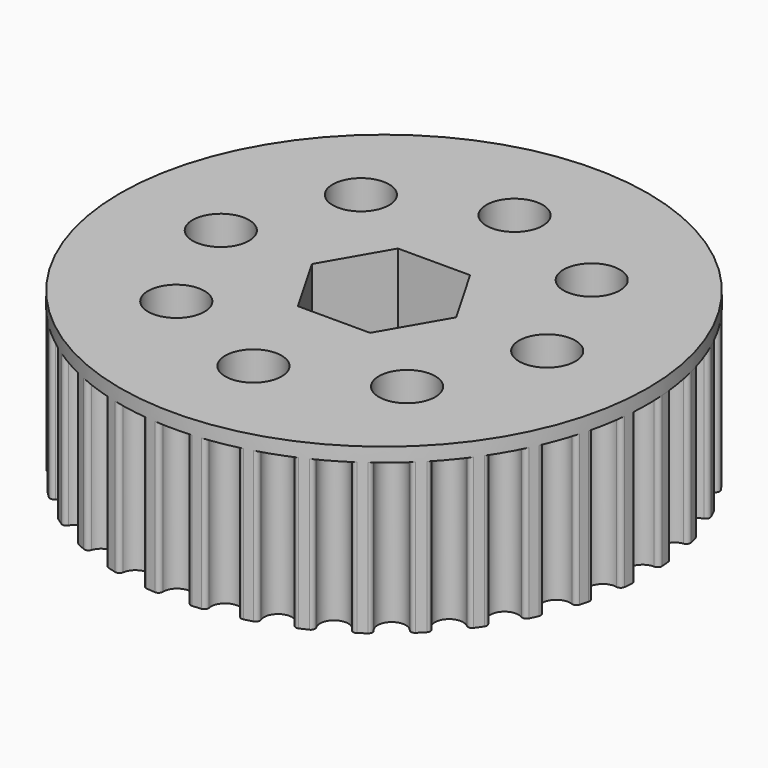
from build123d import *

# Parameters (mm, degrees)
F2_R            = 28.0753897893
F3_DEPTH        = 16
F5_DEPTH        = 16
F5_COPIES_COUNT = 36
F7_R            = 28.0753897893
F8_DEPTH        = 1.5
F9_R            = 3
F10_DEPTH       = 17.501


# Not quite as in the source:
# - a feature of the source that left no trace in its solid (it failed there, or was rolled back) is left out
# - a pattern or mirror of a feature is missing from the dataset's text; its kind, count and spacing are read off the source's solid


with BuildPart() as f3:
    # F2 (on Top) → F3 (new body)
    with BuildSketch(Plane.XY):
        Circle(F2_R)
    extrude(amount=F3_DEPTH)

    # F4 (on face) → F5 (cut, through all)
    with BuildSketch(Plane.XY.offset(16)):
        with BuildLine():
            ThreePointArc((-1.9813235472, 28.0053899959), (-1.6393469358, 27.8824934328), (-1.4996664257, 27.5470222373))
            ThreePointArc((-1.4996664257, 27.5470222373), (0, 26.0153897893), (1.4996664257, 27.5470222373))
            ThreePointArc((1.4996664257, 27.5470222373), (1.6393469358, 27.8824934328), (1.9813235472, 28.0053899959))
            ThreePointArc((1.9813235472, 28.0053899959), (0, 28.0753897893), (-1.9813235472, 28.0053899959))
        make_face()
    f5 = extrude(amount=-F5_DEPTH, mode=Mode.SUBTRACT)

    # F5_copies: F5 ×36 about axis
    f5_copies_axis = Axis((0, 0, 0), (0, 0, 1))
    for i in range(1, F5_COPIES_COUNT):
        add(f5.rotate(f5_copies_axis, i * 360 / F5_COPIES_COUNT), mode=Mode.SUBTRACT)

    # F7 (on face) → F8 (join)
    with BuildSketch(Plane.XY.offset(16)):
        Circle(F7_R)
    extrude(amount=F8_DEPTH)

    # F9 (on face) → F10 (cut, through all)
    with BuildSketch(Plane.XY.offset(17.5)):
        Polygon((-3.8393792901, -6.65), (3.8393792901, -6.65), (7.6787585802, 0), (3.8393792901, 6.65), (-3.8393792901, 6.65), (-7.6787585802, 0), align=None)
        with Locations((12.2772792997, 12.2772792997)):
            Circle(F9_R)
        with Locations((17.3626948946, 0)):
            Circle(F9_R)
        with Locations((12.2772792997, -12.2772792997)):
            Circle(F9_R)
        with Locations((0, -17.3626948946)):
            Circle(F9_R)
        with Locations((-12.2772792997, -12.2772792997)):
            Circle(F9_R)
        with Locations((-17.3626948946, 0)):
            Circle(F9_R)
        with Locations((-12.2772792997, 12.2772792997)):
            Circle(F9_R)
        with Locations((0, 17.3626948946)):
            Circle(F9_R)
    extrude(amount=-F10_DEPTH, mode=Mode.SUBTRACT)


solid = f3.part
